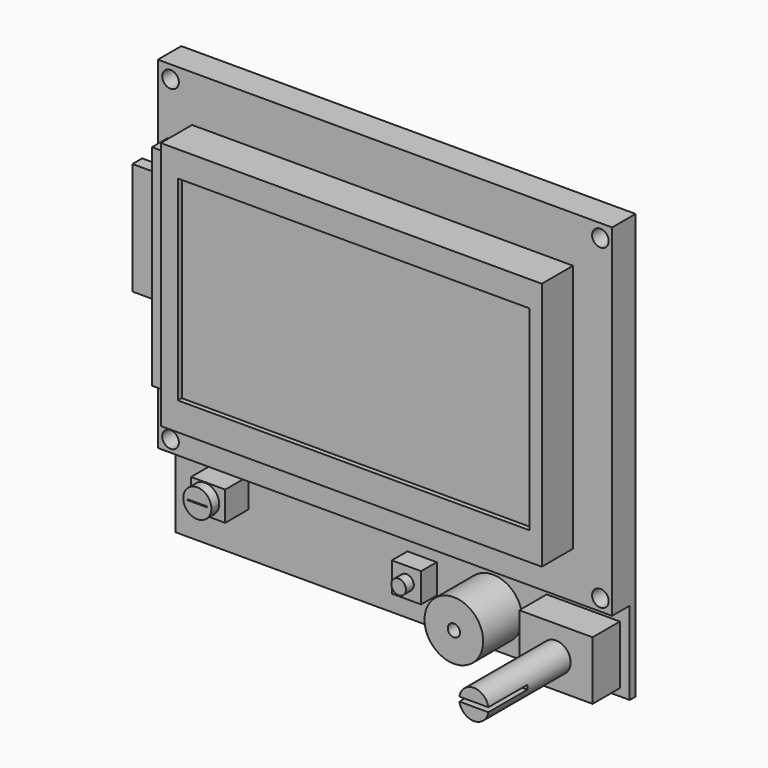
from build123d import *

# Parameters (mm, degrees)
F0_W      = 93
F0_H      = 87
F1_DEPTH  = 6
F2_W      = 78
F2_H      = 51
F3_DEPTH  = 8
F4_W      = 72
F4_H      = 40
F5_DEPTH  = 2
F6_R      = 1.7
F7_DEPTH  = 25
F8_W      = 4
F8_H      = 43
F9_DEPTH  = 5
F10_W     = 93
F10_H     = 17
F11_DEPTH = 4.5
F12_W     = 15
F12_H     = 12
F12_W_2   = 6
F12_H_2   = 6
F12_W_3   = 7
F12_R     = 6
F13_DEPTH = 4
F14_DEPTH = 3
F15_DEPTH = 2
F16_DEPTH = 6
F18_DEPTH = 2
F19_R     = 1.5
F20_DEPTH = 2
F21_R     = 1.25
F22_DEPTH = 3
F23_R     = 3
F24_DEPTH = 21
F25_W     = 6.7849671841
F25_H     = 0.8927487135
F26_DEPTH = 10
F27_W     = 26
F27_H     = 26
F28_DEPTH = 3
F29_W     = 2.5
F29_H     = 23
F30_DEPTH = 22
F31_DEPTH = 32
F32_SIZE  = 4
F33_W     = 20.35
F33_H     = 8.7
F34_DEPTH = 9
F35_DEPTH = 1


with BuildPart() as f1:
    # F0 (on Front) → F1 (new body)
    with BuildSketch(Plane.XZ):
        with Locations((46.5, -43.5)):
            Rectangle(F0_W, F0_H)
    extrude(amount=-F1_DEPTH)

    # F2 (on face) → F3 (join)
    with BuildSketch(Plane.XZ):
        with Locations((46, -35)):
            Rectangle(F2_W, F2_H)
    extrude(amount=F3_DEPTH)

    # F4 (on face) → F5 (cut)
    with BuildSketch(Plane.XZ.offset(8)):
        with Locations((46.5, -34.75)):
            Rectangle(F4_W, F4_H)
    extrude(amount=-F5_DEPTH, mode=Mode.SUBTRACT)

    # F6 (on face) → F7 (cut)
    with BuildSketch(Plane.XZ):
        with Locations((2.6, -2.7)):
            Circle(F6_R)
        with Locations((90.6, -2.7)):
            Circle(F6_R)
        with Locations((90.6, -67.6)):
            Circle(F6_R)
        with Locations((2.6, -67.6)):
            Circle(F6_R)
    extrude(amount=-F7_DEPTH, mode=Mode.SUBTRACT)

    # F8 (on face) → F9 (join)
    with BuildSketch(Plane(origin=(7, 0, 0), x_dir=(0, -1, 0), z_dir=(-1, 0, 0))):
        with Locations((2, -35)):
            Rectangle(F8_W, F8_H)
    extrude(amount=F9_DEPTH)

    # F10 (on face) → F11 (cut)
    with BuildSketch(Plane.XZ):
        with Locations((46.5, -78.5)):
            Rectangle(F10_W, F10_H)
    extrude(amount=-F11_DEPTH, mode=Mode.SUBTRACT)

    # F12 (on face) → F13 (join)
    with BuildSketch(Plane.XZ.offset(-4.5)):
        with Locations((83.5, -79.5)):
            Rectangle(F12_W, F12_H)
        with Locations((50.5, -78)):
            Rectangle(F12_W_2, F12_H_2)
        with Locations((11.5, -75)):
            Rectangle(F12_W_3, F12_H_2)
        with Locations((65, -79.5)):
            Circle(F12_R)
    extrude(amount=F13_DEPTH)

    # F14 (add): a face of the model
    f14_faces = [f1.faces().sort_by_distance(p)[0] for p in [
        (83.5, 0.5, -79.5),
    ]]
    extrude(f14_faces, amount=F14_DEPTH)

    # F15 (add): a face of the model
    f15_faces = [f1.faces().sort_by_distance(p)[0] for p in [
        (11.5, 0.5, -75),
    ]]
    extrude(f15_faces, amount=F15_DEPTH)

    # F16 (add): a face of the model
    f16_faces = [f1.faces().sort_by_distance(p)[0] for p in [
        (65, 0.5, -79.5),
    ]]
    extrude(f16_faces, amount=F16_DEPTH)

    # F17 (on face) → F18 (join)
    with BuildSketch(Plane.XZ.offset(1.5)):
        with BuildLine():
            ThreePointArc((8, -75), (10.8774275169, -77.8774275169), (13.7548550337, -75))
            ThreePointArc((13.7548550337, -75), (10.8774275169, -72.1225724831), (8, -75))
        make_face()
        Polygon((8.8251130655, -75), (8.8251130655, -74.9121382833), (12.8170177341, -74.9121382833), (12.8170177341, -75), (12.8170177341, -75.0878617167), (8.8251130655, -75.0878617167), align=None, mode=Mode.SUBTRACT)
    extrude(amount=F18_DEPTH)

    # F19 (on face) → F20 (join)
    with BuildSketch(Plane.XZ.offset(-0.5)):
        with Locations((50.5, -78)):
            Circle(F19_R)
    extrude(amount=F20_DEPTH)

    # F21 (on face) → F22 (cut)
    with BuildSketch(Plane.XZ.offset(5.5)):
        with Locations((65, -79.5)):
            Circle(F21_R)
    extrude(amount=-F22_DEPTH, mode=Mode.SUBTRACT)

    # F23 (on face) → F24 (join)
    with BuildSketch(Plane.XZ.offset(2.5)):
        with Locations((83.5, -79.5)):
            Circle(F23_R)
    extrude(amount=F24_DEPTH)

    # F25 (on face) → F26 (cut)
    with BuildSketch(Plane.XZ.offset(23.5)):
        with Locations((83.5, -79.5)):
            Rectangle(F25_W, F25_H)
    extrude(amount=-F26_DEPTH, mode=Mode.SUBTRACT)

    # F27 (on face) → F28 (join)
    with BuildSketch(Plane(origin=(0, 6, 0), x_dir=(-1, 0, 0), z_dir=(0, 1, 0))):
        with Locations((-13, -36)):
            Rectangle(F27_W, F27_H)
    extrude(amount=F28_DEPTH)

    # F29 (on face) → F30 (cut)
    with BuildSketch(Plane(origin=(0, 0, 0), x_dir=(0, -1, 0), z_dir=(-1, 0, 0))):
        with Locations((-7.25, -36)):
            Rectangle(F29_W, F29_H)
    extrude(amount=-F30_DEPTH, mode=Mode.SUBTRACT)


with BuildPart() as f31:
    # F31 (new): a face of the model
    f31_faces = [f1.part.faces().sort_by_distance(p)[0] for p in [
        (22, 7.25, -36),
    ]]
    extrude(f31_faces, amount=F31_DEPTH)

    # F32
    f32_edges = [f31.edges().sort_by_distance(p)[0] for p in [
        (22, 7.25, -24.5),
    ]]
    chamfer(f32_edges, length=F32_SIZE)


with BuildPart() as f1_1:
    add(f1.part)

    # F33 (on face) → F34 (join)
    with BuildSketch(Plane(origin=(0, 6, 0), x_dir=(-1, 0, 0), z_dir=(0, 1, 0))):
        with Locations((-62.675, -10.85)):
            Rectangle(F33_W, F33_H)
        with Locations((-32.325, -10.85)):
            Rectangle(F33_W, F33_H)
    extrude(amount=F34_DEPTH)


with BuildPart() as f35:
    # F35 (new): a face of the model
    f35_faces = [f1_1.part.faces().sort_by_distance(p)[0] for p in [
        (46.5, -6, -34.75),
    ]]
    extrude(f35_faces, amount=F35_DEPTH)


solid = Compound([f31.part, f1_1.part, f35.part])
